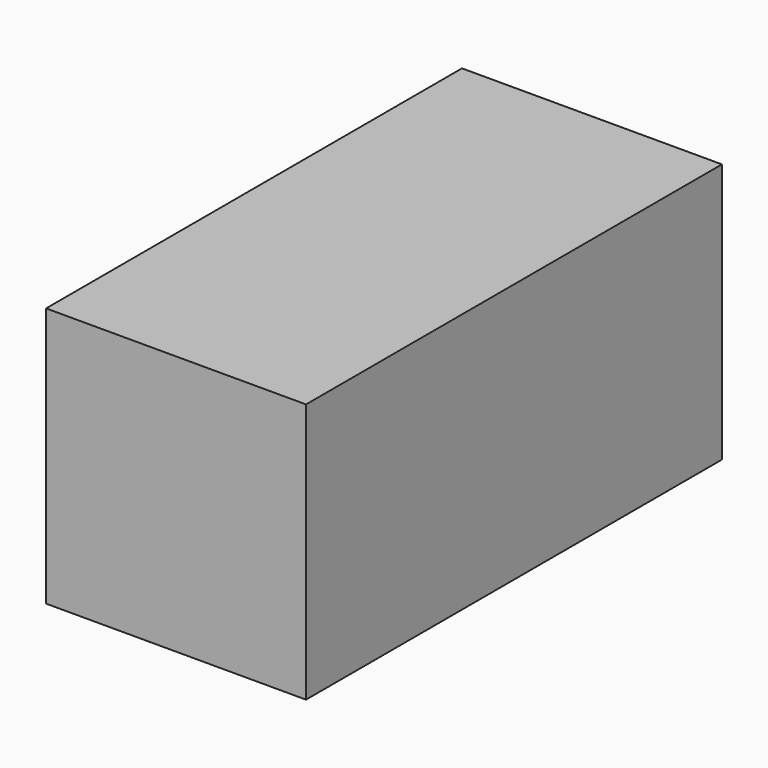
from build123d import *

# Parameters (mm, degrees)
F1_W     = 101.6
F1_H     = 101.6
F2_DEPTH = 101.6


# Not quite as in the source:
# - a variable given as a bare number and used for a length is read in inches; the dataset says mm whatever the document's units were


with BuildPart() as f2:
    # F1 (on Front) → F2 (new body, symmetric)
    with BuildSketch(Plane.XZ):
        Rectangle(F1_W, F1_H)
    extrude(amount=F2_DEPTH, both=True)


solid = f2.part
